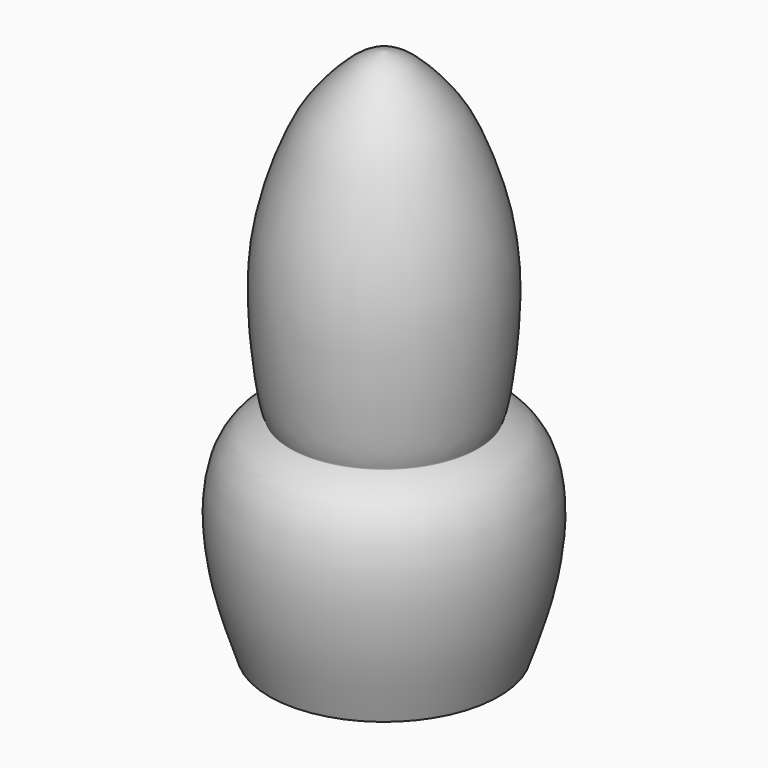
from build123d import *


with BuildPart() as f1:
    # F0 (on Front) → F1 (revolve)
    with BuildSketch(Plane.XZ):
        with BuildLine():
            add(Edge.make_bspline(
                [(-72.7748498321, -166.3143485785), (-77.2057466387, -153.2371327539), (-85.244199491, -129.1212464301), (-89.4079793153, -101.7316628297), (-90.3271827452, -81.9454425783), (-86.9507730364, -55.9463113917), (-73.9682189543, -39.110877653), (-63.7855067332, -34.889111093), (-60.653682964, -33.0155922869), (-58.8688396105, -32.8375153537), (-61.9681986252, -28.4890620391), (-70.171522343, 31.0884947998), (-64.7004266285, 82.2703988998), (-47.9441627473, 126.4512164315), (-36.5226006456, 144.0043904023), (-15.1830007576, 167.3862865224), (-4.3276960868, 169.7625282152), (0, 170.5907136202)],
                knots=[0, 0, 0, 0, 0.0914289313, 0.166474755, 0.2306699906, 0.304113044, 0.369922676, 0.4165800019, 0.4432158616, 0.4580006715, 0.4823040677, 0.5910996965, 0.7018146771, 0.7976382699, 0.8653660634, 0.9445486135, 1, 1, 1, 1], degree=3))
            Line((-72.7748498321, -166.3143485785), (-65.9792870283, -166.3143485785))
            add(Edge.make_bspline(
                [(-65.9792870283, -166.3143485785), (-66.9290410072, -161.7685187143), (-68.691992273, -152.3009907584), (-70.6420646126, -133.187690082), (-56.4017485251, -96.6790049566), (-43.596647439, -94.1249963314), (-42.521855775, -94.3476598161), (-41.5314174374, -94.3078808043), (-41.4739607998, -95.3627091829), (-38.9186895261, -103.7069394197), (-34.1250191238, -121.4228441739), (-31.4236070578, -132.336123076), (-31.2326866704, -133.8637338834), (-30.7375736405, -134.2317885242), (-29.311489218, -134.4866570177), (-14.4240118418, -134.3510872016), (0, -134.2197358608)],
                knots=[0, 0, 0, 0, 0.094974082, 0.209813045, 0.3682203018, 0.4497250124, 0.4746890746, 0.4970085138, 0.5178621736, 0.5902664945, 0.7065017903, 0.7907267702, 0.8183835362, 0.8356078226, 0.8591768806, 1, 1, 1, 1], degree=3))
            Line((0, -134.2197358608), (0, 170.5907136202))
        make_face()
    revolve(axis=Axis((0, 0, 18.1854888797), (0, 0, -1)))


solid = f1.part
